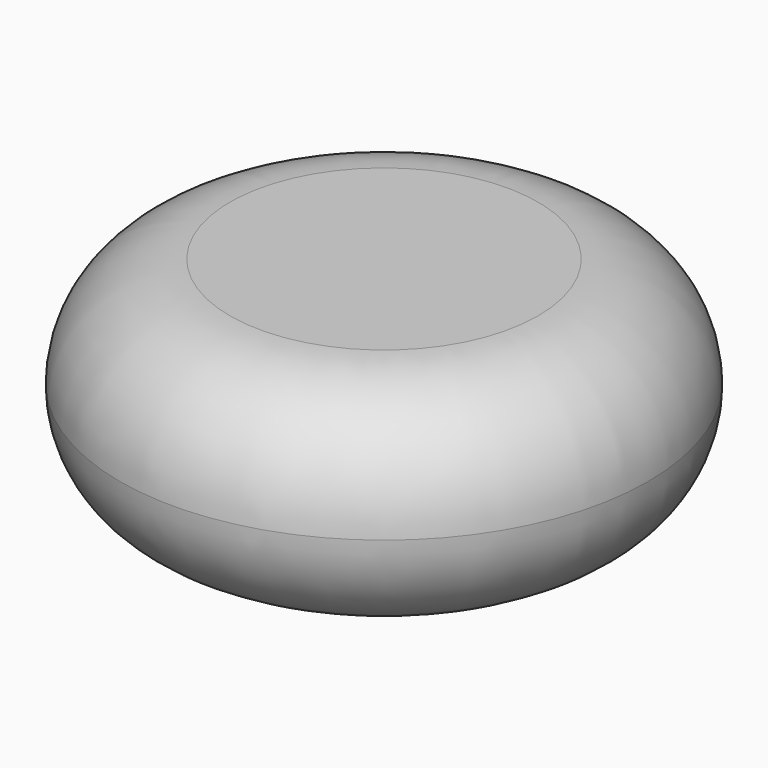
from build123d import *

# Parameters (mm, degrees)
F0_R     = 3
F1_DEPTH = 2.5
F2_R     = 1.24999


# Not quite as in the source:
# - a fillet or chamfer is up to 0.001 mm smaller than in the source, because OpenCascade refuses the exact size


with BuildPart() as f1:
    # F0 (on Top) → F1 (new body)
    with BuildSketch(Plane.XY):
        Circle(F0_R)
    extrude(amount=F1_DEPTH)

    # F2 (radius 1.25 in the source; OpenCascade refuses exactly that, so slightly less here)
    f2_edges = [f1.edges().sort_by_distance(p)[0] for p in [
        (-3, 0, 2.5),
        (-3, 0, 0),
    ]]
    fillet(f2_edges, radius=F2_R)


solid = f1.part
